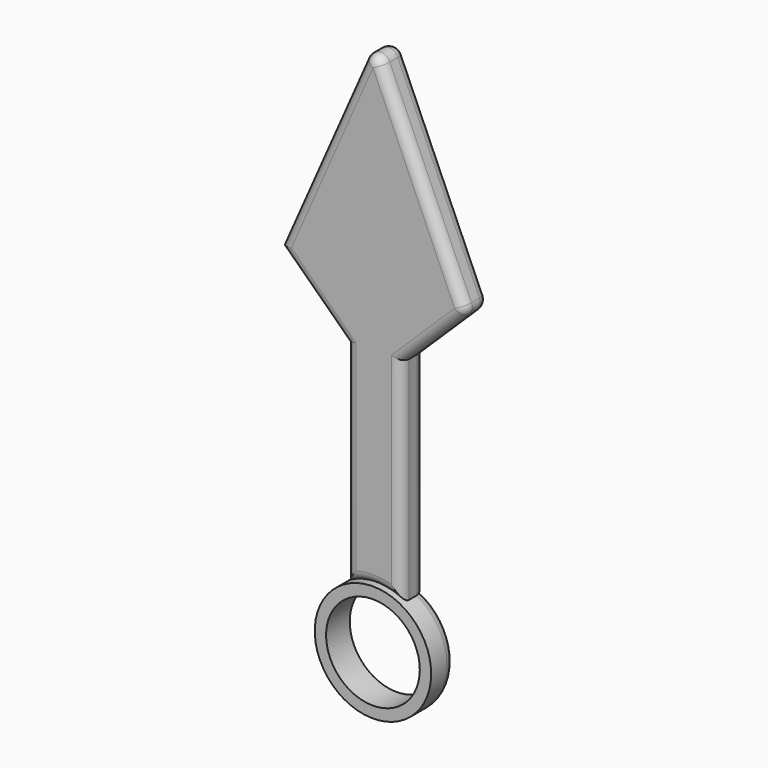
from build123d import *

# Parameters (mm, degrees)
F1_DEPTH = 5
F2_DEPTH = 6
F0_R     = 11.813064162
F0_R_2   = 9.5088348367
F3_R     = 2
F3_2_R   = 2


# Not quite as in the source:
# - a feature of the source that left no trace in its solid (it failed there, or was rolled back) is left out


with BuildPart() as f1:
    # F0 (on Front) → F1 (new body)
    with BuildSketch(Plane.XZ):
        with BuildLine():
            Line((18.9558565617, 32.4459187686), (0, 75.4745528102))
            Line((0, 75.4745528102), (-18.9558584243, 32.4459187686))
            Line((-18.9558584243, 32.4459187686), (-5.4657990113, 19.4210316986))
            Line((-5.4657990113, 19.4210316986), (-5.4657990113, 0))
            Line((-5.4657990113, 0), (-5.4657990113, -23.3750138432))
            ThreePointArc((-5.4657990113, -23.3750138432), (0.1536859635, -22.0490794669), (5.7371167932, -23.5194581672))
            Line((5.7371167932, -23.5194581672), (5.7371167932, 0.0881423131))
            Line((5.7371167932, 0.0881423131), (5.7371167932, 19.5091740117))
            Line((5.7371167932, 19.5091740117), (18.9558565617, 32.4459187686))
        make_face()
    extrude(amount=F1_DEPTH)

    # F0 (on Front) → F2 (join)
    with BuildSketch(Plane.XZ):
        with BuildLine():
            Line((18.9558565617, 32.4459187686), (0, 75.4745528102))
            Line((0, 75.4745528102), (-18.9558584243, 32.4459187686))
            Line((-18.9558584243, 32.4459187686), (-5.4657990113, 19.4210316986))
            Line((-5.4657990113, 19.4210316986), (-5.4657990113, 0))
            Line((-5.4657990113, 0), (-5.4657990113, -23.3750138432))
            ThreePointArc((-5.4657990113, -23.3750138432), (0.1536859635, -22.0490794669), (5.7371167932, -23.5194581672))
            Line((5.7371167932, -23.5194581672), (5.7371167932, 0.0881423131))
            Line((5.7371167932, 0.0881423131), (5.7371167932, 19.5091740117))
            Line((5.7371167932, 19.5091740117), (18.9558565617, 32.4459187686))
        make_face()
    extrude(amount=F2_DEPTH)

    # F3
    f3_edges = [f1.edges().sort_by_distance(p)[0] for p in [
        (9.477928, -6, 53.960236),
        (-9.477929, -6, 53.960236),
        (-12.210829, -6, 25.933475),
        (-5.465799, -6, -1.976991),
        (0.153686, -6, -22.049079),
        (5.737117, -6, -2.005142),
        (12.346487, -6, 25.977546),
        (18.955857, -3, 32.445919),
        (0, -3, 75.474553),
        (9.477928, 0, 53.960236),
        (12.346487, 0, 25.977546),
        (-12.210829, 0, 25.933475),
        (-5.465799, 0, -1.976991),
        (5.737117, 0, -2.005142),
        (-9.477929, 0, 53.960236),
        (0.153686, 0, -22.049079),
    ]]
    fillet(f3_edges, radius=F3_R)


with BuildPart() as f2:
    # F0 (on Front) → F2, piece 2 (new body)
    with BuildSketch(Plane.XZ):
        with Locations((0, -33.9687649328)):
            Circle(F0_R)
        with Locations((0, -33.9687649328)):
            Circle(F0_R_2, mode=Mode.SUBTRACT)
    extrude(amount=F2_DEPTH)

    # F3#2
    f3_2_edges = [f2.edges().sort_by_distance(p)[0] for p in [
        (-11.813064, 0, -33.968765),
    ]]
    fillet(f3_2_edges, radius=F3_2_R)


solid = Compound([f1.part, f2.part])
